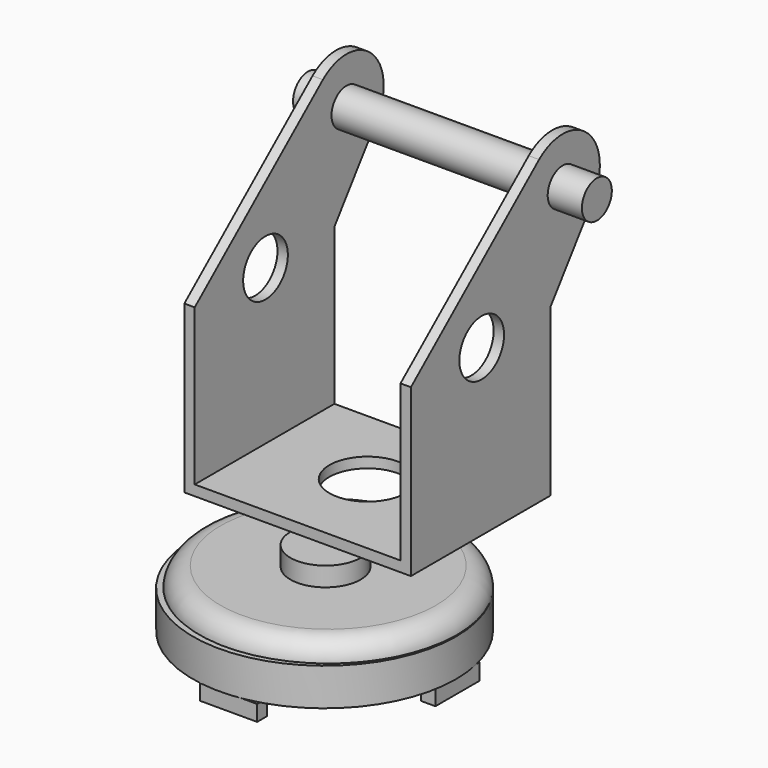
from build123d import *

# Parameters (mm, degrees)
F1_DEPTH       = 50.5
F1_DEPTH_BACK  = 4
F3_START       = -28.11069
F2_R           = 31
F3_DEPTH       = 10.75335
F4_T           = -2.54
F6_START       = -23.50211
F5_R           = 8.452934194
F6_DEPTH       = 12.54557
F8_START       = -32.71926
F7_R           = 31.6455996423
F7_R_2         = 28.4241664141
F8_DEPTH       = 9.01571
F10_START      = -14.77584
F10_DEPTH      = 3.20249
F12_START      = 41.05404
F11_W          = 13.7322936207
F11_H          = 3.7868991494
F12_DEPTH      = 2.93765
F14_START      = -10.76646
F14_DEPTH      = 3.13601
F16_START      = 44.82978
F16_DEPTH      = 3.52112
F18_T          = -2.5
F19_R          = 6.7177835251
F20_DEPTH      = 64.6292769679
F19_R_2        = 4.5
F21_DEPTH      = 61.25
F21_DEPTH_BACK = 8.2255
F22_R          = 9.1649239527
F23_DEPTH      = 25


# Not quite as in the source:
# - a fillet or chamfer that OpenCascade refuses, or shapes differently, is made with other operations: its cross-section is extruded or revolved along the edge and cut away or added
# - a feature names something its author has since deleted; it is built from what else it names


with BuildPart() as f1:
    # F0 (on Right) → F1 (new body, two sides)
    with BuildSketch(Plane.YZ) as f1_sk:
        with BuildLine():
            Line((10.3682326153, 59.2565201223), (-28.1709354445, 26.7167001963))
            Line((-28.1709354445, 26.7167001963), (-28.1709354445, -13.2832998037))
            Line((-28.1709354445, -13.2832998037), (13.8290645555, -13.2832998037))
            Line((13.8290645555, -13.2832998037), (13.8290645555, 26.7167001963))
            Line((13.8290645555, 26.7167001963), (26.480615139, 44.0150722861))
            ThreePointArc((26.480615139, 44.0150722861), (25.1396676432, 58.7347658993), (10.3682326153, 59.2565201223))
        make_face()
    extrude(amount=F1_DEPTH)
    extrude(f1_sk.sketch, amount=-F1_DEPTH_BACK)

    # F18
    f18_openings = [f1.faces().sort_by_distance(p)[0] for p in [
        (23.25, -28.170935, 6.7167),
        (23.25, -8.901351, 42.98661),
        (23.25, 25.139668, 58.734766),
        (23.25, 20.15484, 35.365886),
        (23.25, 13.829065, 6.7167),
    ]]
    offset(amount=F18_T, openings=f18_openings)

    # F19 (on face) → F20 (cut, through all)
    with BuildSketch(Plane.YZ.offset(50.5)):
        with Locations((-6.886796712, 26.4344837213)):
            Circle(F19_R)
    extrude(amount=-F20_DEPTH, mode=Mode.SUBTRACT)

    # F19 (on face) → F21 (join, two sides)
    with BuildSketch(Plane.YZ.offset(50.5)) as f21_sk:
        with Locations((17.4578964769, 50.6140389959)):
            Circle(F19_R_2)
    extrude(amount=-F21_DEPTH)
    extrude(f21_sk.sketch, amount=F21_DEPTH_BACK)

    # F22 (on face) → F23 (cut)
    with BuildSketch(Plane.XY.offset(-10.7832998037)):
        with Locations((22.4927030504, -6.2033818103)):
            Circle(F22_R)
    extrude(amount=-F23_DEPTH, mode=Mode.SUBTRACT)


with BuildPart() as f3:
    # F2 (on Top) → F3 (new body)
    with BuildSketch(Plane.XY.offset(F3_START)):
        with Locations((17.9013703018, -12.2895361856)):
            Circle(F2_R)
    extrude(amount=-F3_DEPTH)

    # F4
    f4_openings = [f3.faces().sort_by_distance(p)[0] for p in [
        (17.90137, -12.289536, -38.86404),
    ]]
    offset(amount=F4_T, openings=f4_openings)

    # F17: fillet of radius 5.08 on 2 edges, made by hand

    # F17_s1 → F17_t2 (revolve, cut)
    with BuildSketch(Plane.XZ.offset(12.2895361856)):
        with BuildLine():
            ThreePointArc((48.9013703018, -33.19069), (47.4134727503, -29.5985875516), (43.8213703018, -28.11069))
            Line((43.8213703018, -28.11069), (43.8213703018, -28.00909))
            Line((43.8213703018, -28.00909), (49.0029703018, -28.00909))
            Line((49.0029703018, -28.00909), (49.0029703018, -33.19069))
            Line((49.0029703018, -33.19069), (48.9013703018, -33.19069))
        make_face()
    revolve(axis=Axis((17.9013703018, -12.2895361856, -28.11069), (0, 0, 1)), mode=Mode.SUBTRACT)

    # F17_s3 → F17_t4 (revolve, cut)
    with BuildSketch(Plane.XZ.offset(12.2895361856)):
        with BuildLine():
            ThreePointArc((48.9013703018, -34.4646309488), (48.2207793531, -37.0046309488), (46.3613703018, -38.86404))
            Line((46.3613703018, -38.86404), (46.4121703018, -38.952028181))
            ThreePointArc((46.4121703018, -38.952028181), (47.6313703018, -38.96564), (48.9013703018, -38.96564))
            Line((48.9013703018, -38.96564), (49.0029703018, -38.86404))
            Line((49.0029703018, -38.86404), (49.0029703018, -34.4646309488))
            Line((49.0029703018, -34.4646309488), (48.9013703018, -34.4646309488))
        make_face()
    revolve(axis=Axis((17.9013703018, -12.2895361856, -38.86404), (0, 0, 1)), mode=Mode.SUBTRACT)


with BuildPart() as f6:
    # F5 (on Top) → F6 (new body)
    with BuildSketch(Plane.XY.offset(F6_START)):
        with Locations((17.773354426, -12.9296155646)):
            Circle(F5_R)
    extrude(amount=-F6_DEPTH)


with BuildPart() as f8:
    # F7 (on Top) → F8 (new body)
    with BuildSketch(Plane.XY.offset(F8_START)):
        with Locations((17.5173226744, -12.9296155646)):
            Circle(F7_R)
        with Locations((17.5173226744, -12.9296155646)):
            Circle(F7_R_2, mode=Mode.SUBTRACT)
    extrude(amount=-F8_DEPTH)

    # F13 (on Right) → F14 (join)
    with BuildSketch(Plane.YZ.offset(F14_START)):
        Polygon((-4.7413306311, -41.4641164243), (-18.1000400335, -41.3919053972), (-18.1000400335, -45.7244589925), (-4.7413306311, -45.7244589925), align=None)
    extrude(amount=-F14_DEPTH)


with BuildPart() as f10:
    # F9 (on Front) → F10 (new body)
    with BuildSketch(Plane.XZ.offset(F10_START)):
        Polygon((26.2270197272, -41.841134429), (12.5101599842, -41.841134429), (12.5101599842, -45.600567013), (24.1948924959, -45.600567013), (26.2270197272, -45.600567013), align=None)
    extrude(amount=-F10_DEPTH)


with BuildPart() as f12:
    # F11 (on Front) → F12 (new body)
    with BuildSketch(Plane.XZ.offset(F12_START)):
        with Locations((19.3067053333, -43.7439270318)):
            Rectangle(F11_W, F11_H)
    extrude(amount=F12_DEPTH)


with BuildPart() as f16:
    # F15 (on Right) → F16 (new body)
    with BuildSketch(Plane.YZ.offset(F16_START)):
        Polygon((-18.1187018752, -45.6302501261), (-4.8111323267, -45.6302501261), (-4.8111323267, -41.7353510857), (-18.1187018752, -41.7894460261), align=None)
    extrude(amount=F16_DEPTH)


solid = Compound([f1.part, f3.part, f6.part, f8.part, f10.part, f12.part, f16.part])
